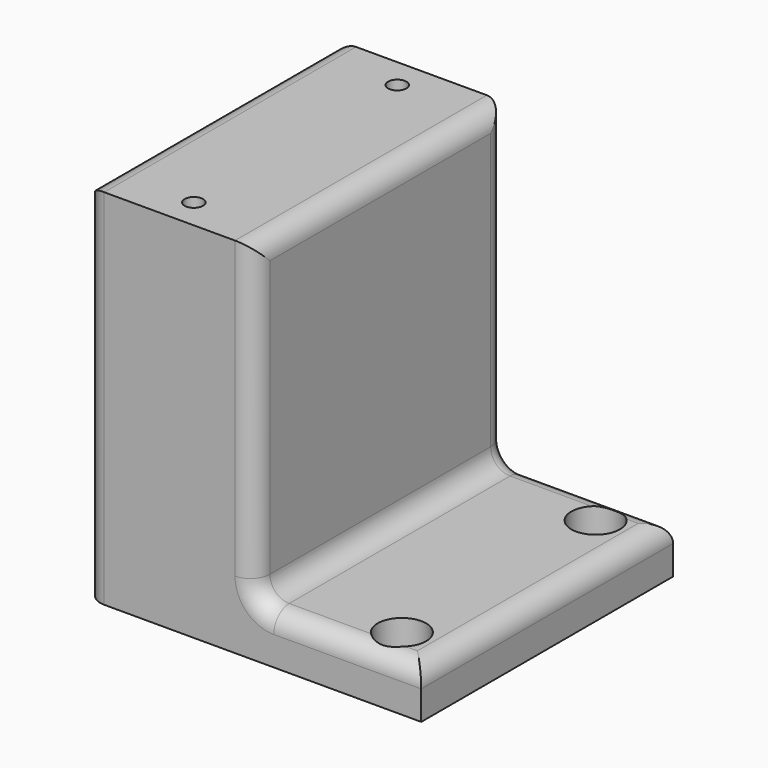
from build123d import *

# Parameters (mm, degrees)
F1_DEPTH       = 82.55
F2_F1_R        = 5.08
F2_F2_R        = 5.08
F4_D           = 4.826
F4_DEPTH       = 25.4
F4_TIP         = 1.4498766737
F6_D           = 6.35
F6_DEPTH       = 25.4
F6_TIP         = 1.9077324654
F8_D           = 6.35
F8_DEPTH       = 25.4
F8_START       = 0.3707141
F8_CBORE_D     = 12.7
F8_CBORE_DEPTH = 6.35
F8_TIP         = 1.9077324654


with BuildPart() as f1:
    # F0 (on Front) → F1 (new body)
    with BuildSketch(Plane.XZ):
        Polygon((0, 95.25), (0, 0), (88.2142, 0), (88.2142, 12.7), (44.45, 12.7), (44.45, 95.25), align=None)
    extrude(amount=F1_DEPTH)

    # F2: fillet of radius 5.08 on 8 edges, made by hand

    # F2_f1
    f2_f1_edges = [f1.edges().sort_by_distance(p)[0] for p in [
        (44.45, -41.275, 12.7),
    ]]
    fillet(f2_f1_edges, radius=F2_F1_R)

    # F2_f2
    f2_f2_edges = [f1.edges().sort_by_distance(p)[0] for p in [
        (44.45, -41.275, 95.25),
        (0, -41.275, 95.25),
        (44.45, -82.55, 56.515),
        (44.45, 0, 56.515),
        (0, -82.55, 47.625),
        (0, 0, 47.625),
        (88.2142, -41.275, 12.7),
        (45.9378975516, 0, 14.1878975516),
        (45.9378975516, -82.55, 14.1878975516),
    ]]
    fillet(f2_f2_edges, radius=F2_F2_R)

    # F4
    with Locations(Plane.XY.offset(95.25)):
        with Locations((22.225, -7.9375), (22.225, -74.6125)):
            Hole(F4_D / 2, depth=F4_DEPTH)
            with Locations((0, 0, -(F4_DEPTH + F4_TIP / 2))):  # 118° drill point
                Cone(0, F4_D / 2, F4_TIP, mode=Mode.SUBTRACT)

    # F6
    with Locations(Plane(origin=(0, 0, 0), x_dir=(1, 0, 0), z_dir=(0, 0, -1))):
        with Locations((12.7, 73.025), (12.7, 9.525)):
            Hole(F6_D / 2, depth=F6_DEPTH)
            with Locations((0, 0, -(F6_DEPTH + F6_TIP / 2))):  # 118° drill point
                Cone(0, F6_D / 2, F6_TIP, mode=Mode.SUBTRACT)

    # F8
    # its depths count from where the whole tool has entered the part; down to there all is cleared
    with Locations(Plane.XY.offset(12.7).offset(-F8_START)):
        with Locations((75.5142, -9.525), (75.5142, -73.025)):
            CounterBoreHole(F8_D / 2, F8_CBORE_D / 2, F8_CBORE_DEPTH, depth=F8_DEPTH)
            with Locations((0, 0, -(F8_DEPTH + F8_TIP / 2))):  # 118° drill point
                Cone(0, F8_D / 2, F8_TIP, mode=Mode.SUBTRACT)


solid = f1.part
